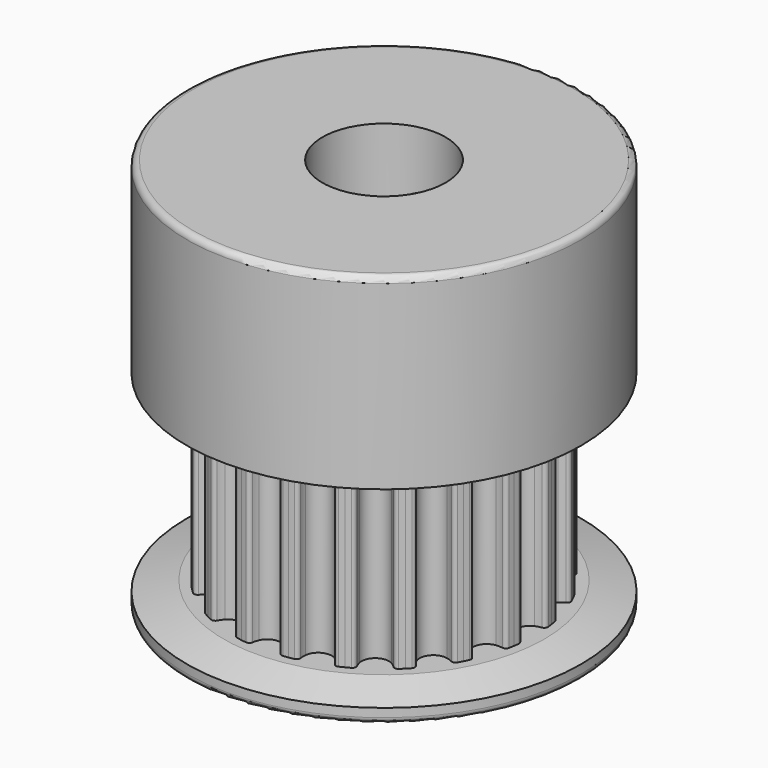
from build123d import *

# Parameters (mm, degrees)
F3_DEPTH    = 3.5
F4_COUNT    = 20
F5_R        = 8
F6_DEPTH    = 1
F7_R        = 8
F8_DEPTH    = 1
F9_R        = 8
F10_DEPTH   = 7
F11_R       = 2.5
F12_DEPTH   = 16.001
F13_R       = 1.75
F14_DEPTH   = 8.001
F15_R       = 1.75
F16_DEPTH   = 8.0010001
F17_SIZE2   = 0.4019237886
F17_SIZE    = 1.5
F17_2_SIZE2 = 0.4019237886
F17_2_SIZE  = 1.5
F18_R       = 0.25


# Not quite as in the source:
# - a feature names something its author has since deleted; it is built from what else it names


with BuildPart() as f3:
    # F2 (on Top) → F3 (new body, symmetric)
    with BuildSketch(Plane.XY):
        with BuildLine():
            ThreePointArc((0.5072317048, 5.6927824446), (0.3024954694, 5.4527213714), (0, 5.3630400697))
            ThreePointArc((0, 5.3630400697), (-0.3024954694, 5.4527213714), (-0.5072317048, 5.6927824446))
            ThreePointArc((-0.5072317048, 5.6927824446), (-0.5520948337, 5.8145502635), (-0.5808117717, 5.9411023854))
            ThreePointArc((-0.5808117717, 5.9411023854), (-0.6387574174, 6.037333963), (-0.7472774352, 6.0663446529))
            ThreePointArc((-0.7472774352, 6.0663446529), (-0.8518447388, 6.0525466999), (-0.9561583811, 6.0369464271))
            Line((-0.9561583811, 6.0369464271), (0, 0))
            Line((0, 0), (0.9561583811, 6.0369464271))
            ThreePointArc((0.9561583811, 6.0369464271), (0.8518447388, 6.0525466999), (0.7472774352, 6.0663446529))
            ThreePointArc((0.7472774352, 6.0663446529), (0.6387574174, 6.037333963), (0.5808117717, 5.9411023854))
            ThreePointArc((0.5808117717, 5.9411023854), (0.5520948337, 5.8145502635), (0.5072317048, 5.6927824446))
        make_face()
    extrude(amount=F3_DEPTH, both=True)

    # F4: F3 ×20 about axis
    f4_axis = Axis((0, 0, 0), (0, 0, -1))


with BuildPart() as f3_1:
    add(f3.part)
    for i in range(1, F4_COUNT):
        add(f3.part.rotate(f4_axis, i * 360 / F4_COUNT))

    # F5 (on face) → F6 (join)
    with BuildSketch(Plane(origin=(0, 0, -3.5), x_dir=(1, 0, 0), z_dir=(0, 0, -1))):
        Circle(F5_R)
    extrude(amount=F6_DEPTH)

    # F7 (on face) → F8 (join)
    with BuildSketch(Plane.XY.offset(3.5)):
        Circle(F7_R)
    extrude(amount=F8_DEPTH)

    # F9 (on face) → F10 (join)
    with BuildSketch(Plane.XY.offset(4.5)):
        Circle(F9_R)
    extrude(amount=F10_DEPTH)

    # F11 (on face) → F12 (cut, through all)
    with BuildSketch(Plane.XY.offset(11.5)):
        Circle(F11_R)
    extrude(amount=-F12_DEPTH, mode=Mode.SUBTRACT)

    # F13 (on Front) → F14 (cut, through all)
    with BuildSketch(Plane.XZ):
        with Locations((0, 7.5)):
            Circle(F13_R)
    extrude(amount=-F14_DEPTH, mode=Mode.SUBTRACT)

    # F15 (on Right) → F16 (cut, through all)
    with BuildSketch(Plane.YZ):
        with Locations((0, 7.5)):
            Circle(F15_R)
    extrude(amount=-F16_DEPTH, mode=Mode.SUBTRACT)

    # F17
    f17_edges = [f3_1.edges().sort_by_distance(p)[0] for p in [
        (-8, 0, -3.5),
    ]]
    f17_side = f3_1.faces().sort_by_distance((-7.773726, 0, -3.5))[0]
    chamfer(f17_edges, length=F17_SIZE, length2=F17_SIZE2, reference=f17_side)

    # F17#2
    f17_2_edges = [f3_1.edges().sort_by_distance(p)[0] for p in [
        (-8, 0, 3.5),
    ]]
    f17_2_side = f3_1.faces().sort_by_distance((-7.773726, 0, 3.5))[0]
    chamfer(f17_2_edges, length=F17_2_SIZE, length2=F17_2_SIZE2, reference=f17_2_side)

    # F18
    f18_edges = [f3_1.edges().sort_by_distance(p)[0] for p in [
        (-8, 0, 11.5),
        (-8, 0, -4.5),
    ]]
    fillet(f18_edges, radius=F18_R)


solid = f3_1.part
